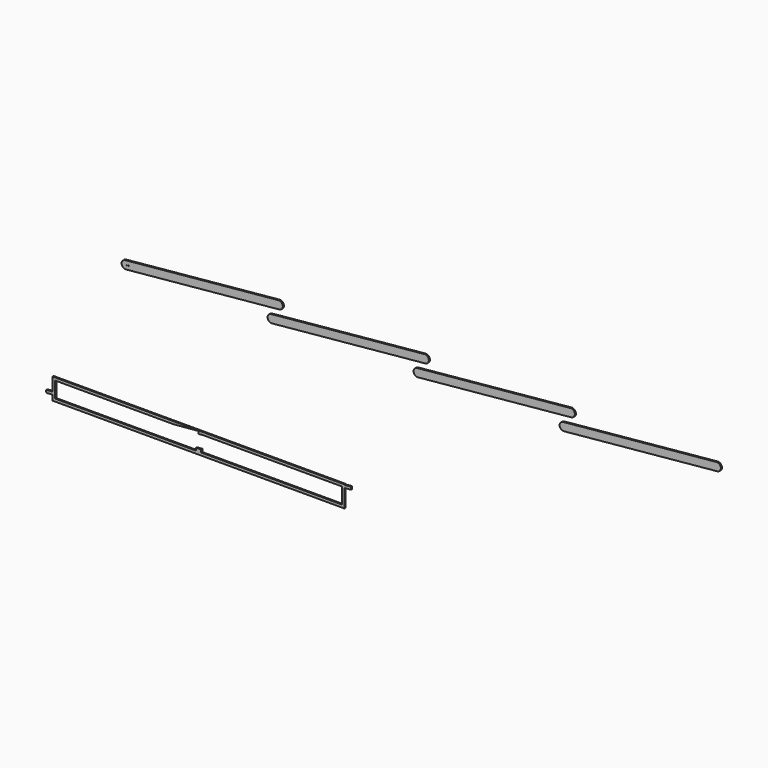
from build123d import *

# Parameters (mm, degrees)
F1_DEPTH = 50


# Not quite as in the source:
# - ends of sketch curves that miss each other by under 0.0002 mm in the source are joined


with BuildPart() as f1:
    # F0 (on Front) → F1 (new body)
    with BuildSketch(Plane.XZ):
        with BuildLine():
            Line((-3.5807e-05, -3.4109e-06), (-14.224173738, 149.3240532582))
            ThreePointArc((-14.224173738, 149.3240532582), (-149.3240566691, -14.224137931), (14.224102124, -149.32406008))
            Line((14.224102124, -149.32406008), (-3.5807e-05, -3.4109e-06))
        make_face()
        with BuildLine():
            Line((5759.6393866078, 699.3240566691), (-14.224173738, 149.3240532582))
            ThreePointArc((-14.224173738, 149.3240532582), (95.5300548118, 115.6460489063), (149.3240566691, 14.224137931))
            Line((149.3240566691, 14.224137931), (5624.5394678697, 535.775862069))
            ThreePointArc((5624.5394678697, 535.775862069), (5658.2174870863, 645.5300686774), (5759.6393866078, 699.3240566691))
        make_face()
        with BuildLine():
            ThreePointArc((149.3240566691, 14.224137931), (95.5300548118, 115.6460489063), (-14.224173738, 149.3240532582))
            Line((-14.224173738, 149.3240532582), (-3.5807e-05, -3.4109e-06))
            Line((-3.5807e-05, -3.4109e-06), (149.3240566691, 14.224137931))
        make_face()
        with BuildLine():
            Line((-3.5807e-05, -3.4109e-06), (14.224102124, -149.32406008))
            ThreePointArc((14.224102124, -149.32406008), (110.9811139758, -100.9118047639), (150, 0))
            Line((150, 0), (-3.5807e-05, -3.4109e-06))
        make_face()
        with BuildLine():
            ThreePointArc((150, 0), (110.9811139758, -100.9118047639), (14.224102124, -149.32406008))
            Line((14.224102124, -149.32406008), (1581.818181818, 0))
            Line((1581.818181818, 0), (150, 0))
        make_face()
        with BuildLine():
            Line((5624.5394678697, 535.775862069), (149.3240566691, 14.224137931))
            ThreePointArc((149.3240566691, 14.224137931), (149.8309188725, 7.1200947899), (150, 0))
            Line((150, 0), (1581.818181818, 0))
            Line((1581.818181818, 0), (5788.0876624699, 400.6759433309))
            ThreePointArc((5788.0876624699, 400.6759433309), (5678.3334558614, 434.3539625474), (5624.5394678697, 535.775862069))
        make_face()
        with BuildLine():
            Line((5773.8635245388, 550), (5759.6393866078, 699.3240566691))
            ThreePointArc((5759.6393866078, 699.3240566691), (5658.2174870863, 645.5300686774), (5624.5394678697, 535.775862069))
            Line((5624.5394678697, 535.775862069), (5773.8635245388, 550))
        make_face()
        with BuildLine():
            ThreePointArc((5923.8635245388, 550), (5874.7753159964, 660.9811260748), (5759.6393866078, 699.3240566691))
            Line((5759.6393866078, 699.3240566691), (5773.8635245388, 550))
            Line((5773.8635245388, 550), (5788.0876624699, 400.6759433309))
            ThreePointArc((5788.0876624699, 400.6759433309), (5884.8446506136, 449.0882085424), (5923.8635245388, 550))
        make_face()
        with BuildLine():
            Line((5773.8635245388, 550), (5624.5394678697, 535.775862069))
            ThreePointArc((5624.5394678697, 535.775862069), (5678.3334558614, 434.3539625474), (5788.0876624699, 400.6759433309))
            Line((5788.0876624699, 400.6759433309), (5773.8635245388, 550))
        make_face()
    extrude(amount=F1_DEPTH)


with BuildPart() as f1b:
    # F0 (on Front) → F1, piece 2 (new body)
    with BuildSketch(Plane.XZ):
        with BuildLine():
            ThreePointArc((5485.7757801252, 149.3240488634), (5389.0188462368, 100.9117610063), (5350, 0))
            Line((5350, 0), (5650, 0))
            ThreePointArc((5650, 0), (5600.9117610063, 110.9811537632), (5485.7757801252, 149.3240488634))
        make_face()
        with BuildLine():
            Line((5650, 0), (5350, 0))
            ThreePointArc((5350, 0), (5399.0881771331, -110.9810975152), (5514.224053409, -149.3240647204))
            ThreePointArc((5514.224053409, -149.3240647204), (5610.9810975152, -100.9118228669), (5650, 0))
        make_face()
        with BuildLine():
            Line((11259.6394721102, 699.3240648138), (5485.7757801252, 149.3240488634))
            ThreePointArc((5485.7757801252, 149.3240488634), (5600.9117610063, 110.9811537632), (5650, 0))
            ThreePointArc((5650, 0), (5610.9810975152, -100.9118228669), (5514.224053409, -149.3240647204))
            Line((5514.224053409, -149.3240647204), (11288.087745394, 400.67595123))
            ThreePointArc((11288.087745394, 400.67595123), (11124.5394677469, 535.7758633581), (11259.6394721102, 699.3240648138))
        make_face()
        with BuildLine():
            ThreePointArc((11423.8635245388, 550), (11374.7753477701, 660.9810971839), (11259.6394721102, 699.3240648138))
            ThreePointArc((11259.6394721102, 699.3240648138), (11124.5394677469, 535.7758633581), (11288.087745394, 400.67595123))
            ThreePointArc((11288.087745394, 400.67595123), (11384.8446786333, 449.088239358), (11423.8635245388, 550))
        make_face()
    extrude(amount=F1_DEPTH)


with BuildPart() as f1c:
    # F0 (on Front) → F1, piece 3 (new body)
    with BuildSketch(Plane.XZ):
        with BuildLine():
            ThreePointArc((11014.224137931, -149.3240566691), (11110.9811260748, -100.9117914576), (11150, 0))
            ThreePointArc((11150, 0), (11100.9117914575, 110.9811260748), (10985.775862069, 149.3240566691))
            Line((10985.775862069, 149.3240566691), (11014.224137931, -149.3240566691))
        make_face()
        with BuildLine():
            ThreePointArc((10985.775862069, 149.3240566691), (11100.9117914575, 110.9811260748), (11150, 0))
            ThreePointArc((11150, 0), (11110.9811260748, -100.9117914576), (11014.224137931, -149.3240566691))
            Line((11014.224137931, -149.3240566691), (16788.0876624699, 400.6759433309))
            ThreePointArc((16788.0876624699, 400.6759433309), (16624.5394678697, 535.775862069), (16759.6393866078, 699.3240566691))
            Line((16759.6393866078, 699.3240566691), (10985.775862069, 149.3240566691))
        make_face()
        with BuildLine():
            Line((11014.224137931, -149.3240566691), (10985.775862069, 149.3240566691))
            ThreePointArc((10985.775862069, 149.3240566691), (10850.6759433309, -14.224137931), (11014.224137931, -149.3240566691))
        make_face()
        with BuildLine():
            Line((16788.0876624699, 400.6759433309), (16759.6393866078, 699.3240566691))
            ThreePointArc((16759.6393866078, 699.3240566691), (16624.5394678697, 535.775862069), (16788.0876624699, 400.6759433309))
        make_face()
        with BuildLine():
            ThreePointArc((16923.8635245388, 550), (16874.7753159964, 660.9811260748), (16759.6393866078, 699.3240566691))
            Line((16759.6393866078, 699.3240566691), (16788.0876624699, 400.6759433309))
            ThreePointArc((16788.0876624699, 400.6759433309), (16884.8446506136, 449.0882085424), (16923.8635245388, 550))
        make_face()
    extrude(amount=F1_DEPTH)


with BuildPart() as f1d:
    # F0 (on Front) → F1, piece 4 (new body)
    with BuildSketch(Plane.XZ):
        with BuildLine():
            ThreePointArc((16514.2240542685, -149.3240646385), (16610.9810978056, -100.9118225475), (16650, 0))
            ThreePointArc((16650, 0), (16600.9117603676, 110.9811543439), (16485.7757784065, 149.3240486997))
            ThreePointArc((16485.7757784065, 149.3240486997), (16350.6759433309, -14.224137931), (16514.2240542685, -149.3240646385))
        make_face()
        with BuildLine():
            ThreePointArc((16485.7757784065, 149.3240486997), (16600.9117603676, 110.9811543439), (16650, 0))
            ThreePointArc((16650, 0), (16610.9810978056, -100.9118225475), (16514.2240542685, -149.3240646385))
            Line((16514.2240542685, -149.3240646385), (22288.0877459291, 400.6759512809))
            ThreePointArc((22288.0877459291, 400.675951281), (22124.5394678697, 535.775862069), (22259.639470067, 699.3240646191))
            Line((22259.639470067, 699.3240646192), (16485.7757784065, 149.3240486997))
        make_face()
        with BuildLine():
            ThreePointArc((22423.8635245388, 550), (22374.7753470108, 660.9810978743), (22259.639470067, 699.3240646191))
            ThreePointArc((22259.639470067, 699.3240646191), (22124.5394678697, 535.775862069), (22288.0877459291, 400.675951281))
            ThreePointArc((22288.0877459291, 400.675951281), (22384.8446788141, 449.0882395569), (22423.8635245388, 550))
        make_face()
    extrude(amount=F1_DEPTH)


with BuildPart() as f1e:
    # F0 (on Front) → F1, piece 5 (new body)
    with BuildSketch(Plane.XZ):
        Polygon((2750, -4617.8705309245), (2750, -4600), (-2750, -4600), (-2750, -5099.0581803171), (-2650, -5090.3093139645), (-2650, -4700), (1811.2558728689, -4700), align=None)
        Polygon((2954.2611031453, -4600), (2750, -4600), (2750, -4617.8705309245), align=None)
        Polygon((2954.2611031453, -4600), (2750, -4617.8705309245), (2750, -4718.2525146788), (2850, -4709.5036483262), (2850, -4700), (2958.6271974359, -4700), (2992.1681885505, -4697.065543514), (2983.676053874, -4600), align=None)
        Polygon((2983.4526142757, -4597.4460737049), (2954.2611031453, -4600), (2983.676053874, -4600), align=None)
        Polygon((-2650, -5090.3093139645), (-2750, -5099.0581803171), (-2750, -5199.4401640714), (-2650, -5190.6912977188), align=None)
        Polygon((-2750, -5199.4401640714), (-2750, -5099.0581803171), (-2993.7155742748, -5120.3805301908), (-2985, -5220), align=None)
        Polygon((8250, -4600), (2983.676053874, -4600), (2992.1681885505, -4697.065543514), (2958.6271974359, -4700), (7311.2558728688, -4700), (8250, -4617.8705309245), align=None)
        Polygon((-2650, -5190.6912977188), (-2750, -5199.4401640714), (-2750, -5400), (2750, -5400), (2750, -5199.4401640714), (2650, -5208.189030424), (2650, -5300), (-2650, -5300), align=None)
        Polygon((2850, -5190.6912977188), (2750, -5199.4401640714), (2750, -5400), (8250, -5400), (8250, -4718.2525146788), (8150, -4727.0013810314), (8150, -5300), (2850, -5300), align=None)
        Polygon((8483.4526142757, -4597.4460737049), (8250, -4617.8705309245), (8250, -4718.2525146788), (8492.1681885505, -4697.065543514), align=None)
        Polygon((8250, -4718.2525146788), (8250, -4617.8705309245), (7311.2558728688, -4700), (8150, -4700), (8150, -4727.0013810314), align=None)
    extrude(amount=F1_DEPTH)


solid = Compound([f1.part, f1b.part, f1c.part, f1d.part, f1e.part])
